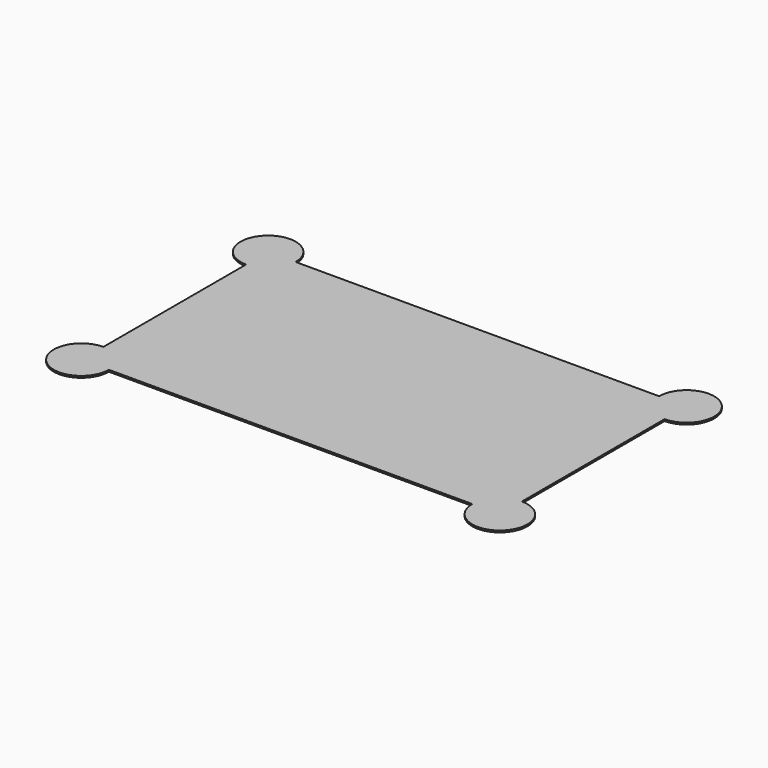
from build123d import *

# Parameters (mm, degrees)
F0_W     = 190
F0_H     = 106
F1_DEPTH = 0.8
F2_R     = 12.5
F3_DEPTH = 0.8


# Not quite as in the source:
# - a feature names something its author has since deleted; it is built from what else it names


with BuildPart() as f1:
    # F0 (on Top) → F1 (new body)
    with BuildSketch(Plane.XY):
        with Locations((-95, 53)):
            Rectangle(F0_W, F0_H)
    extrude(amount=F1_DEPTH)

    # F2 (on face) → F3 (join)
    with BuildSketch(Plane(origin=(0, 0, 0), x_dir=(1, 0, 0), z_dir=(0, 0, -1))):
        Circle(F2_R)
        with Locations((-190, 0)):
            Circle(F2_R)
        with Locations((-190, -106)):
            Circle(F2_R)
        with Locations((0, -106)):
            Circle(F2_R)
    extrude(amount=-F3_DEPTH)


solid = f1.part
